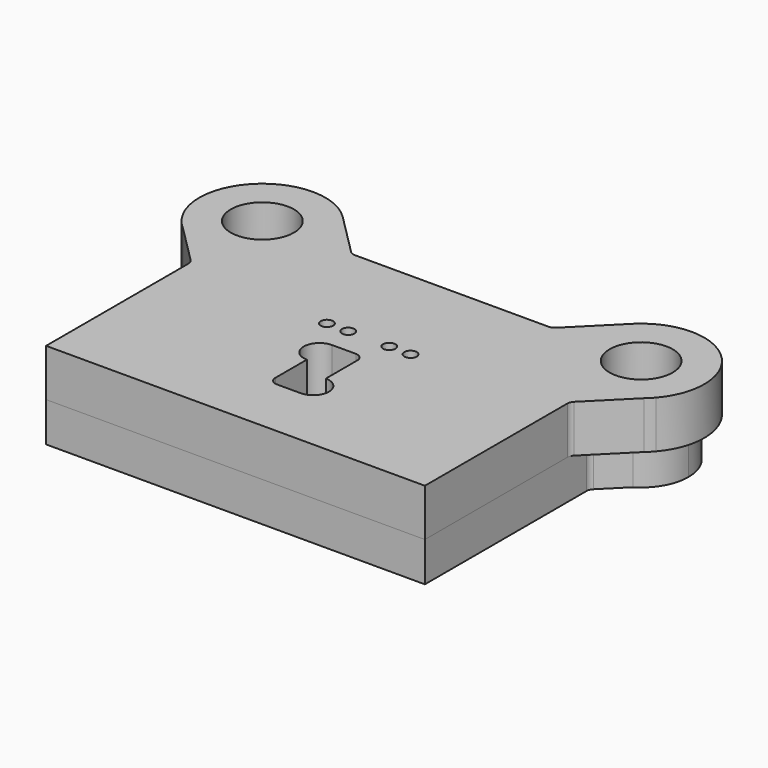
from build123d import *

# Parameters (mm, degrees)
F0_R      = 25.4
F1_DEPTH  = 31.75
F4_R      = 25.4
F5_DEPTH  = 38.1
F7_DEPTH  = 25.4
F9_R      = 5
F10_DEPTH = 25.4
F12_DEPTH = 38.1


with BuildPart() as f1:
    # F0 (on Top) → F1 (new body)
    with BuildSketch(Plane.XY):
        with BuildLine():
            Line((-152.4, 53.9033839703), (-152.4, -108.7667216295))
            Line((-152.4, -108.7667216295), (152.4, -108.7667216295))
            Line((152.4, -108.7667216295), (152.4, 53.9033839703))
            ThreePointArc((152.4, 53.9033839703), (152.8833649686, 56.3334237658), (154.2598719395, 58.3935120309))
            Line((154.2598719395, 58.3935120309), (171.9035763614, 76.0372164528))
            ThreePointArc((171.9035763614, 76.0372164528), (125.6457900901, 81.6406778321), (119.4044321158, 127.8167216295))
            Line((119.4044321158, 127.8167216295), (102.2143040553, 110.626593569))
            ThreePointArc((102.2143040553, 110.626593569), (100.1542157903, 109.2500865981), (97.7241759947, 108.7667216295))
            Line((97.7241759947, 108.7667216295), (-97.7241759947, 108.7667216295))
            ThreePointArc((-97.7241759947, 108.7667216295), (-100.1542157903, 109.2500865981), (-102.2143040553, 110.626593569))
            Line((-102.2143040553, 110.626593569), (-119.4044321158, 127.8167216295))
            ThreePointArc((-119.4044321158, 127.8167216295), (-115.5982260184, 118.6277272479), (-114.3, 108.7667216295))
            ThreePointArc((-114.3, 108.7667216295), (-125.4592316368, 81.8259532663), (-152.4, 70.6667216295))
            Line((-152.4, 70.6667216295), (-152.4, 53.9033839703))
        make_face()
        with BuildLine():
            ThreePointArc((-171.9035763614, 76.0372164528), (-162.5147380778, 72.0338742907), (-152.4, 70.6667216295))
            ThreePointArc((-152.4, 70.6667216295), (-125.4592316368, 81.8259532663), (-114.3, 108.7667216295))
            ThreePointArc((-114.3, 108.7667216295), (-115.5982260184, 118.6277272479), (-119.4044321158, 127.8167216295))
            ThreePointArc((-119.4044321158, 127.8167216295), (-179.1542099099, 135.8927654269), (-171.9035763614, 76.0372164528))
        make_face()
        with Locations((-152.4, 108.7667216295)):
            Circle(F0_R, mode=Mode.SUBTRACT)
        with BuildLine():
            ThreePointArc((119.4044321158, 127.8167216295), (125.6457900901, 81.6406778321), (171.9035763614, 76.0372164528))
            ThreePointArc((171.9035763614, 76.0372164528), (185.5262453303, 89.9448760687), (190.5, 108.7667216295))
            ThreePointArc((190.5, 108.7667216295), (162.2610056184, 145.5684956111), (119.4044321158, 127.8167216295))
        make_face()
        with Locations((152.4, 108.7667216295)):
            Circle(F0_R, mode=Mode.SUBTRACT)
        with BuildLine():
            ThreePointArc((-154.2598719395, 58.3935120309), (-152.8833649686, 56.3334237658), (-152.4, 53.9033839703))
            Line((-152.4, 53.9033839703), (-152.4, 70.6667216295))
            ThreePointArc((-152.4, 70.6667216295), (-162.5147380778, 72.0338742907), (-171.9035763614, 76.0372164528))
            Line((-171.9035763614, 76.0372164528), (-154.2598719395, 58.3935120309))
        make_face()
    extrude(amount=F1_DEPTH)


with BuildPart() as f2_1:
    # F2: copy of F1
    add(f1.part)


with BuildPart() as f5:
    # F4 (on face) → F5 (new body)
    with BuildSketch(Plane.XY.offset(31.75)):
        with BuildLine():
            Line((-152.4, -108.7667216295), (152.4, -108.7667216295))
            Line((152.4, -108.7667216295), (152.4, 34.487204177))
            ThreePointArc((152.4, 34.487204177), (152.8833649686, 36.9172439725), (154.2598719395, 38.9773322375))
            Line((154.2598719395, 38.9773322375), (185.5948326386, 70.3122929367))
            Line((185.5948326386, 70.3122929367), (190.8544286929, 75.5718889909))
            ThreePointArc((190.8544286929, 75.5718889909), (187.3817017696, 145.6031240231), (117.2645696221, 145.4565231029))
            Line((117.2645696221, 145.4565231029), (115.7101985266, 143.9021520075))
            Line((115.7101985266, 143.9021520075), (82.4346400881, 110.626593569))
            ThreePointArc((82.4346400881, 110.626593569), (80.3745518231, 109.2500865981), (77.9445120276, 108.7667216295))
            Line((77.9445120276, 108.7667216295), (-77.9445120276, 108.7667216295))
            ThreePointArc((-77.9445120276, 108.7667216295), (-80.3745518231, 109.2500865981), (-82.4346400881, 110.626593569))
            Line((-82.4346400881, 110.626593569), (-115.7101985266, 143.9021520075))
            Line((-115.7101985266, 143.9021520075), (-117.2645696221, 145.4565231029))
            ThreePointArc((-117.2645696221, 145.4565231029), (-187.3817017696, 145.6031240231), (-190.8544286929, 75.5718889909))
            Line((-190.8544286929, 75.5718889909), (-185.5948326386, 70.3122929367))
            Line((-185.5948326386, 70.3122929367), (-154.2598719395, 38.9773322375))
            ThreePointArc((-154.2598719395, 38.9773322375), (-152.8833649686, 36.9172439725), (-152.4, 34.487204177))
            Line((-152.4, 34.487204177), (-152.4, -108.7667216295))
        make_face()
        with Locations((-152.4, 108.7667216295)):
            Circle(F4_R, mode=Mode.SUBTRACT)
        with Locations((152.4, 108.7667216295)):
            Circle(F4_R, mode=Mode.SUBTRACT)
        with BuildLine():
            Line((190.8544286929, 75.5718889909), (185.5948326386, 70.3122929367))
            ThreePointArc((185.5948326386, 70.3122929367), (188.3210244843, 72.8456971453), (190.8544286929, 75.5718889909))
        make_face()
        with BuildLine():
            ThreePointArc((-190.8544286929, 75.5718889909), (-188.3210244843, 72.8456971453), (-185.5948326386, 70.3122929367))
            Line((-185.5948326386, 70.3122929367), (-190.8544286929, 75.5718889909))
        make_face()
        with BuildLine():
            Line((115.7101985266, 143.9021520075), (117.2645696221, 145.4565231029))
            ThreePointArc((117.2645696221, 145.4565231029), (116.4789755157, 144.6877461138), (115.7101985266, 143.9021520075))
        make_face()
        with BuildLine():
            ThreePointArc((-115.7101985266, 143.9021520075), (-116.4789755157, 144.6877461138), (-117.2645696221, 145.4565231029))
            Line((-117.2645696221, 145.4565231029), (-115.7101985266, 143.9021520075))
        make_face()
    extrude(amount=F5_DEPTH)

    # F9 (on face) → F10 (cut)
    with BuildSketch(Plane.XY.offset(69.85)):
        with Locations((-33.655, 25.2733201705)):
            Circle(F9_R)
        with Locations((-16.51, 25.2733201705)):
            Circle(F9_R)
        with Locations((16.51, 25.2733201705)):
            Circle(F9_R)
        with Locations((33.655, 25.2733201705)):
            Circle(F9_R)
    extrude(amount=-F10_DEPTH, mode=Mode.SUBTRACT)

    # F11 (on face) → F12 (cut, through all)
    with BuildSketch(Plane.XY.offset(69.85)):
        with BuildLine():
            ThreePointArc((12.6999875243, -59.1816798295), (25.3999875243, -46.4816798295), (12.6999875243, -33.7816798295))
            Line((12.6999875243, -33.7816798295), (12.6999875243, -2.0316798295))
            ThreePointArc((12.6999875243, -2.0316798295), (10.8401155849, 2.458448231), (6.3499875243, 4.3183201705))
            Line((6.3499875243, 4.3183201705), (-12.7000124757, 4.3183201705))
            ThreePointArc((-12.7000124757, 4.3183201705), (-25.4000124757, -8.3816798295), (-12.7000124757, -21.0816798295))
            Line((-12.7000124757, -21.0816798295), (-12.7000124757, -52.8316798295))
            ThreePointArc((-12.7000124757, -52.8316798295), (-10.8401405362, -57.3218078901), (-6.3500124757, -59.1816798295))
            Line((-6.3500124757, -59.1816798295), (12.6999875243, -59.1816798295))
        make_face()
    extrude(amount=-F12_DEPTH, mode=Mode.SUBTRACT)


with BuildPart() as f1_1:
    add(f1.part)

    # F6 (on face) → F7 (cut)
    with BuildSketch(Plane(origin=(0, 0, 0), x_dir=(1, 0, 0), z_dir=(0, 0, -1))):
        with BuildLine():
            Line((-25.4, 71.8816688296), (-25.4, 67.1191688296))
            ThreePointArc((-25.4, 67.1191688296), (-22.0324039546, 68.5140727842), (-20.6375, 71.8816688296))
            Line((-20.6375, 71.8816688296), (-25.4, 71.8816688296))
        make_face()
        with BuildLine():
            ThreePointArc((-20.6375, 71.8816688296), (-28.7675960454, 75.249264875), (-25.4, 67.1191688296))
            Line((-25.4, 67.1191688296), (-25.4, 71.8816688296))
            Line((-25.4, 71.8816688296), (-20.6375, 71.8816688296))
        make_face()
        with BuildLine():
            Line((25.4, 71.8816688296), (25.4, 67.1191688296))
            ThreePointArc((25.4, 67.1191688296), (28.7675960454, 68.5140727842), (30.1625, 71.8816688296))
            ThreePointArc((30.1625, 71.8816688296), (25.4, 76.6441688296), (20.6375, 71.8816688296))
            Line((20.6375, 71.8816688296), (25.4, 71.8816688296))
        make_face()
        with BuildLine():
            ThreePointArc((20.6375, 71.8816688296), (22.0324039546, 68.5140727842), (25.4, 67.1191688296))
            Line((25.4, 67.1191688296), (25.4, 71.8816688296))
            Line((25.4, 71.8816688296), (20.6375, 71.8816688296))
        make_face()
        with BuildLine():
            ThreePointArc((-20.6375, -17.0183311704), (-22.0324039546, -13.650735125), (-25.4, -12.2558311704))
            Line((-25.4, -12.2558311704), (-25.4, -17.0183311704))
            Line((-25.4, -17.0183311704), (-20.6375, -17.0183311704))
        make_face()
        with BuildLine():
            Line((-25.4, -17.0183311704), (-25.4, -12.2558311704))
            ThreePointArc((-25.4, -12.2558311704), (-28.7675960454, -20.3859272158), (-20.6375, -17.0183311704))
            Line((-20.6375, -17.0183311704), (-25.4, -17.0183311704))
        make_face()
        with BuildLine():
            Line((25.4, -17.0183311704), (25.4, -12.2558311704))
            ThreePointArc((25.4, -12.2558311704), (22.0324039546, -13.650735125), (20.6375, -17.0183311704))
            Line((20.6375, -17.0183311704), (25.4, -17.0183311704))
        make_face()
        with BuildLine():
            ThreePointArc((30.1625, -17.0183311704), (28.7675960454, -13.650735125), (25.4, -12.2558311704))
            Line((25.4, -12.2558311704), (25.4, -17.0183311704))
            Line((25.4, -17.0183311704), (20.6375, -17.0183311704))
            ThreePointArc((20.6375, -17.0183311704), (25.4, -21.7808311704), (30.1625, -17.0183311704))
        make_face()
    extrude(amount=-F7_DEPTH, mode=Mode.SUBTRACT)


solid = Compound([f5.part, f1_1.part])
